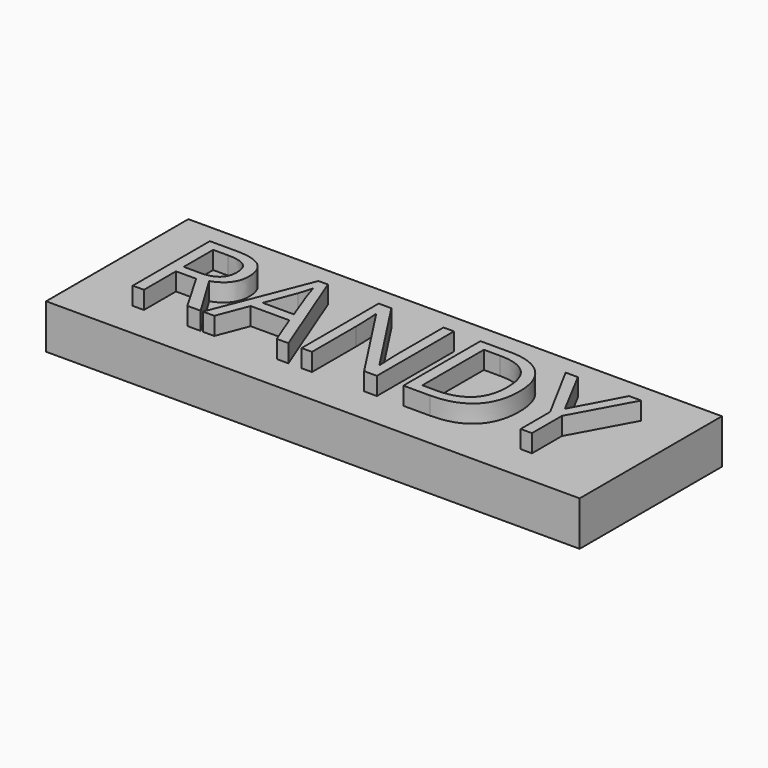
from build123d import *

# Parameters (mm, degrees)
F0_W         = 60
F0_H         = 20
F1_DEPTH     = 5
F2_TEXT_SIZE = 15.1795455624
F3_DEPTH     = 2


# Not quite as in the source:
# - Text() gives the source's letters only with a copy of the font that has no kerning and outlines rounded to 1/6400 em; it was checked with that copy


with BuildPart() as f1:
    # F0 (on Top) → F1 (new body)
    with BuildSketch(Plane.XY):
        Rectangle(F0_W, F0_H)
    extrude(amount=F1_DEPTH)

    # F2 (on face) → F3 (join)
    with BuildSketch(Plane.XY.offset(5)):
        with Locations((-25, -5.9292728049)):
            Text('RANDY', F2_TEXT_SIZE, font='Open Sans', text_align=(TextAlign.LEFT, TextAlign.BOTTOM))
    extrude(amount=F3_DEPTH)


solid = f1.part
